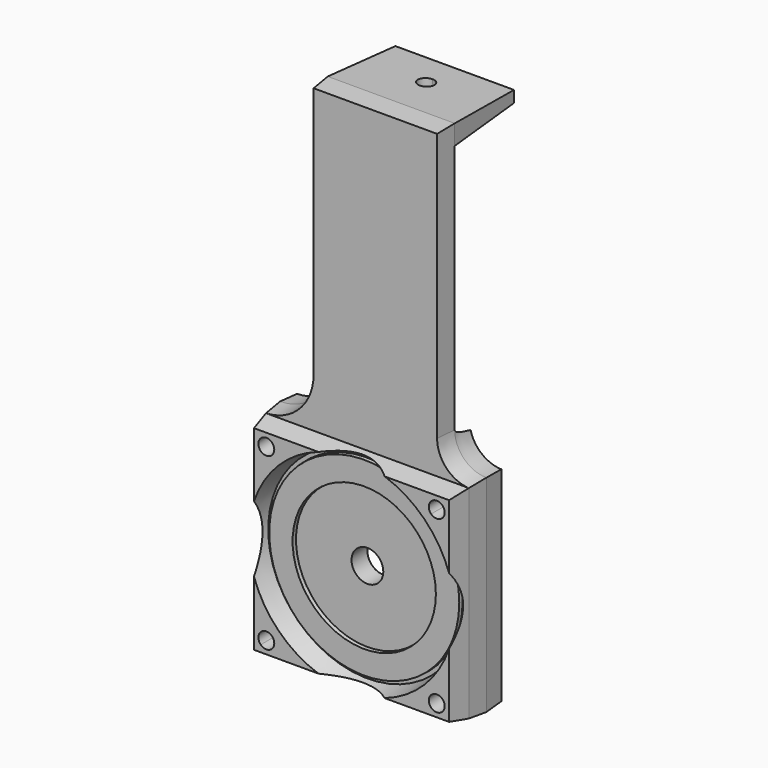
from build123d import *

# Parameters (mm, degrees)
F1_DEPTH                 = 7.9375
DRAFT_F1_DRAFTED_ANGLE   = 5
F2_W                     = 50.8
F2_H                     = 7.9375
F3_DEPTH                 = 31.75
DRAFT_F3_DRAFTED_ANGLE   = 3
F4_W                     = 12.7
F4_H                     = 82.55
F5_DEPTH                 = 7.9375
F6_R                     = 254
F7_DEPTH                 = 25.4
DRAFT_F7_DRAFTED_ANGLE   = -3
F9_DEPTH                 = 1.5875
DRAFT_F9_DRAFTED_ANGLE   = 3
DRAFT_F9_2_DRAFTED_ANGLE = 3
F10_R                    = 6.35
F11_DEPTH                = 39.6885
F12_R                    = 38.1
F12_R_2                  = 28.575
F13_DEPTH                = 1.5875
F13_TAPER                = 3
F14_R                    = 39.6875
F15_DEPTH                = 7.9375
F15_TAPER                = 11
F16_R                    = 3.175
F17_DEPTH                = 9.525
F18_R                    = 2.413
F18_R_2                  = 3.175
F19_DEPTH                = 25.4
F21_DEPTH                = 203.201
F23_DEPTH                = 12.7


# Not quite as in the source:
# - an extrude with a draft is written as a straight extrude whose walls are then drafted


with BuildPart() as f1:
    # F0 (on Front) → F1 (new body)
    with BuildSketch(Plane.XZ):
        Polygon((19.05, 101.6), (19.05, 82.55), (69.85, 82.55), (69.85, 95.25), (69.85, 203.2), (19.05, 203.2), align=None)
        Polygon((0, 82.55), (0, 0), (82.55, 0), (82.55, 82.55), (69.85, 82.55), (19.05, 82.55), align=None)
        with BuildLine():
            Line((69.85, 82.55), (82.55, 82.55))
            ThreePointArc((82.55, 82.55), (73.5697438789, 86.2697438789), (69.85, 95.25))
            Line((69.85, 95.25), (69.85, 82.55))
        make_face()
        with BuildLine():
            ThreePointArc((19.05, 101.6), (13.4703841816, 88.1296158184), (0, 82.55))
            Line((0, 82.55), (19.05, 82.55))
            Line((19.05, 82.55), (19.05, 101.6))
        make_face()
    extrude(amount=F1_DEPTH)

    # draft_F1_drafted
    draft_f1_drafted_walls = [f1.faces().sort_by_distance(p)[0] for p in [
        (0, -5.2916666667, 41.275),
        (41.275, -5.2916666667, 0),
        (82.55, -5.2916666667, 41.275),
        (73.5697438789, -5.2916666667, 86.2697438789),
        (69.85, -5.2916666667, 149.225),
        (44.45, -5.2916666667, 203.2),
        (19.05, -5.2916666667, 152.4),
        (13.4703841816, -5.2916666667, 88.1296158184),
    ]]
    draft(draft_f1_drafted_walls, neutral_plane=Plane.XZ, angle=DRAFT_F1_DRAFTED_ANGLE)


with BuildPart() as f3_drafted:
    # F2 (on face) → F3 (new body)
    with BuildSketch(Plane(origin=(0, 0, 0), x_dir=(-1, 0, 0), z_dir=(0, 1, 0))):
        with Locations((-44.45, 199.23125)):
            Rectangle(F2_W, F2_H)
    extrude(amount=F3_DEPTH)

    # draft_F3_drafted
    draft_f3_drafted_walls = [f3_drafted.faces().sort_by_distance(p)[0] for p in [
        (19.05, 21.1666666667, 199.23125),
        (44.45, 21.1666666667, 203.2),
        (69.85, 21.1666666667, 199.23125),
        (44.45, 21.1666666667, 195.2625),
    ]]
    draft(draft_f3_drafted_walls, neutral_plane=Plane(origin=(0, 0, 0), x_dir=(-1, 0, 0), z_dir=(0, 1, 0)), angle=DRAFT_F3_DRAFTED_ANGLE)


with BuildPart() as f1_1:
    add(f1.part)

    # join_F3_drafted: union F3_drafted
    add(f3_drafted.part)

    # F4 (on face) → F5 (join)
    with BuildSketch(Plane(origin=(0, 0, 0), x_dir=(-1, 0, 0), z_dir=(0, 1, 0))):
        with BuildLine():
            ThreePointArc((-69.85, 95.25), (-73.5697438789, 86.2697438789), (-82.55, 82.55))
            Line((-82.55, 82.55), (-69.85, 82.55))
            Line((-69.85, 82.55), (-69.85, 95.25))
        make_face()
        with Locations((-76.2, 41.275)):
            Rectangle(F4_W, F4_H)
        with Locations((-6.35, 41.275)):
            Rectangle(F4_W, F4_H)
        with BuildLine():
            Line((-12.7, 82.55), (0, 82.55))
            ThreePointArc((0, 82.55), (-6.7974608102, 83.8040165618), (-12.7, 87.4009683429))
            Line((-12.7, 87.4009683429), (-12.7, 82.55))
        make_face()
    extrude(amount=F5_DEPTH)


with BuildPart() as f7_drafted:
    # F6 (on face) → F7 (new body)
    with BuildSketch(Plane(origin=(0, 0, 0), x_dir=(-1, 0, 0), z_dir=(0, 1, 0))):
        with Locations((-82.55, 0)):
            Circle(F6_R)
        with BuildLine():
            Line((0, 0), (-12.7, 0))
            Line((-12.7, 0), (-69.85, 0))
            Line((-69.85, 0), (-82.55, 0))
            Line((-82.55, 0), (-82.55, 82.55))
            ThreePointArc((-82.55, 82.55), (-73.5697438789, 86.2697438789), (-69.85, 95.25))
            Line((-69.85, 95.25), (-69.85, 195.2625))
            Line((-69.85, 195.2625), (-69.85, 203.2))
            Line((-69.85, 203.2), (-19.05, 203.2))
            Line((-19.05, 203.2), (-19.05, 195.2625))
            Line((-19.05, 195.2625), (-19.05, 101.6))
            ThreePointArc((-19.05, 101.6), (-17.3901912008, 93.8228700667), (-12.7, 87.4009683429))
            ThreePointArc((-12.7, 87.4009683429), (-6.7974608102, 83.8040165618), (0, 82.55))
            Line((0, 82.55), (0, 0))
        make_face(mode=Mode.SUBTRACT)
    extrude(amount=F7_DEPTH)

    # draft_F7_drafted
    draft_f7_drafted_walls = [f7_drafted.faces().sort_by_distance(p)[0] for p in [
        (336.55, 16.9333333333, 0),
        (19.05, 16.9333333333, 152.4),
        (44.45, 16.9333333333, 203.2),
        (69.85, 16.9333333333, 149.225),
        (73.5697438789, 16.9333333333, 86.2697438789),
        (82.55, 16.9333333333, 41.275),
        (41.275, 16.9333333333, 0),
        (0, 16.9333333333, 41.275),
        (13.4703841816, 16.9333333333, 88.1296158184),
    ]]
    draft(draft_f7_drafted_walls, neutral_plane=Plane(origin=(0, 0, 0), x_dir=(-1, 0, 0), z_dir=(0, 1, 0)), angle=DRAFT_F7_DRAFTED_ANGLE)


with BuildPart() as f1_2:
    add(f1_1.part)

    # join_F7_drafted: cut F7_drafted
    add(f7_drafted.part, mode=Mode.SUBTRACT)


with BuildPart() as f9_drafted:
    # F8 (on face) → F9 (new body)
    with BuildSketch(Plane(origin=(0, 0, 0), x_dir=(-1, 0, 0), z_dir=(0, 1, 0))):
        Polygon((-12.7, 0), (0, 0), (0, 82.55), (-25.4, 82.55), (-25.4, 0), align=None)
    extrude(amount=F9_DEPTH)

    # draft_F9_drafted
    draft_f9_drafted_walls = [f9_drafted.faces().sort_by_distance(p)[0] for p in [
        (12.7, 1.0583333333, 0),
        (12.7, 1.0583333333, 82.55),
        (25.4, 1.0583333333, 41.275),
        (0, 1.0583333333, 41.275),
    ]]
    draft(draft_f9_drafted_walls, neutral_plane=Plane(origin=(0, 0, 0), x_dir=(-1, 0, 0), z_dir=(0, 1, 0)), angle=DRAFT_F9_DRAFTED_ANGLE)


with BuildPart() as f1_3:
    add(f1_2.part)

    # join_F9_drafted: union F9_drafted
    add(f9_drafted.part)


with BuildPart() as f9_2_drafted:
    # F8 (on face) → F9, piece 2 (new body)
    with BuildSketch(Plane(origin=(0, 0, 0), x_dir=(-1, 0, 0), z_dir=(0, 1, 0))):
        Polygon((-69.85, 0), (-63.5, 0), (-63.5, 82.55), (-82.55, 82.55), (-82.55, 0), align=None)
    extrude(amount=F9_DEPTH)

    # draft_F9_2_drafted
    draft_f9_2_drafted_walls = [f9_2_drafted.faces().sort_by_distance(p)[0] for p in [
        (73.025, 1.0583333333, 0),
        (73.025, 1.0583333333, 82.55),
        (82.55, 1.0583333333, 41.275),
        (63.5, 1.0583333333, 41.275),
    ]]
    draft(draft_f9_2_drafted_walls, neutral_plane=Plane(origin=(0, 0, 0), x_dir=(-1, 0, 0), z_dir=(0, 1, 0)), angle=DRAFT_F9_2_DRAFTED_ANGLE)


with BuildPart() as f1_4:
    add(f1_3.part)

    # join_F9_2_drafted: union F9_2_drafted
    add(f9_2_drafted.part)

    # F10 (on face) → F11 (cut, through all)
    with BuildSketch(Plane.XZ.offset(7.9375)):
        with Locations((41.275, 41.2840069672)):
            Circle(F10_R)
    extrude(amount=-F11_DEPTH, mode=Mode.SUBTRACT)

    # F12 (on face) → F13 (join)
    with BuildSketch(Plane.XZ.offset(7.9375)):
        with Locations((41.275, 41.2840069672)):
            Circle(F12_R)
        with Locations((41.275, 41.2840069672)):
            Circle(F12_R_2, mode=Mode.SUBTRACT)
    extrude(amount=F13_DEPTH, taper=F13_TAPER)

    # F14 (on face) → F15 (join)
    with BuildSketch(Plane.XZ.offset(7.9375)):
        Polygon((81.8555587333, 81.8735726677), (0.6944412667, 81.8677747767), (0.6944412667, 0.6944412667), (81.8555587333, 0.6944412667), align=None)
        with Locations((41.275, 41.2840069672)):
            Circle(F14_R, mode=Mode.SUBTRACT)
    extrude(amount=F15_DEPTH, taper=F15_TAPER)

    # F16 (on face) → F17 (cut)
    with BuildSketch(Plane(origin=(0, 7.9375, 0), x_dir=(-1, 0, 0), z_dir=(0, 1, 0))):
        with Locations((-76.2, 22.225)):
            Circle(F16_R)
        with Locations((-76.2, 60.325)):
            Circle(F16_R)
        with Locations((-6.35, 60.325)):
            Circle(F16_R)
        with Locations((-6.35, 22.225)):
            Circle(F16_R)
    extrude(amount=-F17_DEPTH, mode=Mode.SUBTRACT)

    # F18 (on Right) → F19 (cut)
    with BuildSketch(Plane.YZ):
        with Locations((3.8735, 69.85)):
            Circle(F18_R)
        with Locations((3.8735, 12.7)):
            Circle(F18_R)
        with Locations((3.8735, 41.275)):
            Circle(F18_R_2)
    extrude(amount=F19_DEPTH, mode=Mode.SUBTRACT)

    # F20 (on Top) → F21 (cut, through all)
    with BuildSketch(Plane.XY):
        with BuildLine():
            Line((44.45, 20.6375), (44.45, 14.2875))
            ThreePointArc((44.45, 14.2875), (46.6950640303, 15.2174359697), (47.625, 17.4625))
            ThreePointArc((47.625, 17.4625), (46.6950640303, 19.7075640303), (44.45, 20.6375))
        make_face()
        with BuildLine():
            ThreePointArc((44.45, 20.6375), (41.275, 17.4625), (44.45, 14.2875))
            Line((44.45, 14.2875), (44.45, 20.6375))
        make_face()
    extrude(amount=F21_DEPTH, mode=Mode.SUBTRACT)

    # F22 (on face) → F23 (cut)
    with BuildSketch(Plane.XZ.offset(15.875)):
        with BuildLine():
            ThreePointArc((10.3568594887, 75.384481558), (8.3962836808, 78.3180457522), (4.9358838152, 77.6286335747))
            Line((4.9358838152, 77.6286335747), (9.4278351622, 73.1403295413))
            ThreePointArc((9.4278351622, 73.1403295413), (10.115423683, 74.1700573659), (10.3568594887, 75.384481558))
        make_face()
        with BuildLine():
            Line((9.4278351622, 73.1403295413), (4.9358838152, 77.6286335747))
            ThreePointArc((4.9358838152, 77.6286335747), (4.937707472, 73.1385058845), (9.4278351622, 73.1403295413))
        make_face()
        with BuildLine():
            ThreePointArc((77.6134829058, 77.6320559156), (73.1233548798, 77.6326126786), (73.1227981168, 73.1424846526))
            Line((73.1227981168, 73.1424846526), (77.6134829058, 77.6320559156))
        make_face()
        with BuildLine():
            Line((77.6134829058, 77.6320559156), (73.1227981168, 73.1424846526))
            ThreePointArc((73.1227981168, 73.1424846526), (76.5829785452, 72.4538774445), (78.5431405113, 75.3872702841))
            ThreePointArc((78.5431405113, 75.3872702841), (78.3015333508, 76.6021083181), (77.6134829058, 77.6320559156))
        make_face()
        with BuildLine():
            Line((73.1197334269, 9.4224099754), (77.6123143648, 4.9347361329))
            ThreePointArc((77.6123143648, 4.9347361329), (78.2996732647, 5.9643546304), (78.5410238958, 7.1785730541))
            ThreePointArc((78.5410238958, 7.1785730541), (76.5802423196, 10.112222423), (73.1197334269, 9.4224099754))
        make_face()
        with BuildLine():
            ThreePointArc((73.1197334269, 9.4224099754), (73.1221869746, 4.9322825852), (77.6123143648, 4.9347361329))
            Line((77.6123143648, 4.9347361329), (73.1197334269, 9.4224099754))
        make_face()
        with BuildLine():
            Line((4.9388241401, 4.9336007729), (9.4332951597, 9.4193816698))
            ThreePointArc((9.4332951597, 9.4193816698), (4.9431692015, 9.4237267311), (4.9388241401, 4.9336007729))
        make_face()
        with BuildLine():
            ThreePointArc((10.3610596499, 7.1764912213), (10.1199647049, 8.3900917026), (9.4332951597, 9.4193816698))
            Line((9.4332951597, 9.4193816698), (4.9388241401, 4.9336007729))
            ThreePointArc((4.9388241401, 4.9336007729), (8.3996601312, 4.2425861663), (10.3610596499, 7.1764912213))
        make_face()
    extrude(amount=-F23_DEPTH, mode=Mode.SUBTRACT)


solid = f1_4.part
